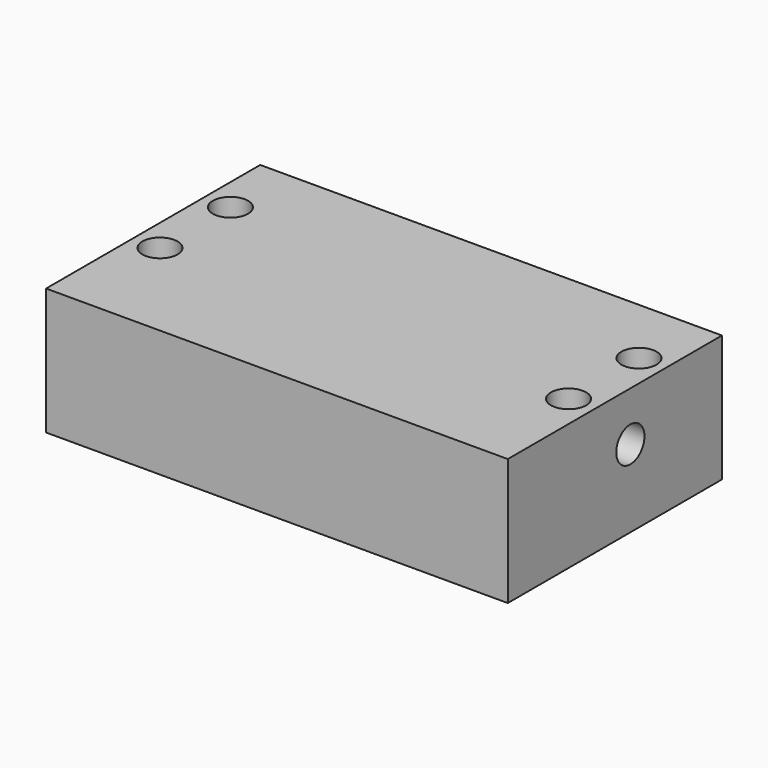
from build123d import *

# Parameters (mm, degrees)
F0_W     = 33.2994
F0_H     = 19.304
F1_DEPTH = 4.572
F2_R     = 1.27
F3_DEPTH = 2.54
F5_D     = 1.778
F5_DEPTH = 2.54
F5_TIP   = 0.5341650903
F8_R     = 1.27
F9_DEPTH = 9.145


# Not quite as in the source:
# - a pattern or mirror of a feature is missing from the dataset's text; its kind, count and spacing are read off the source's solid


with BuildPart() as f1:
    # F0 (on Top) → F1 (new body, symmetric)
    with BuildSketch(Plane.XY):
        Rectangle(F0_W, F0_H)
    extrude(amount=F1_DEPTH, both=True)

    # F2 (on face) → F3 (cut)
    with BuildSketch(Plane(origin=(-16.6497, 0, 0), x_dir=(0, -1, 0), z_dir=(-1, 0, 0))):
        with Locations((-1.397, 1.016)):
            Circle(F2_R)
    f3 = extrude(amount=-F3_DEPTH, mode=Mode.SUBTRACT)

    # F3_copies: F3 across plane
    add(f3.mirror(Plane(origin=(0, 0, 0), x_dir=(0, 0, 1), z_dir=(1, 0, 0))), mode=Mode.SUBTRACT)

    # F5
    with Locations(Plane(origin=(0, 0, -4.572), x_dir=(1, 0, 0), z_dir=(0, 0, -1))):
        with Locations((10.9347, -7.112), (10.9347, 7.112), (-10.9347, -7.112), (-10.9347, 7.112)):
            Hole(F5_D / 2, depth=F5_DEPTH)
            with Locations((0, 0, -(F5_DEPTH + F5_TIP / 2))):  # 118° drill point
                Cone(0, F5_D / 2, F5_TIP, mode=Mode.SUBTRACT)

    # F8 (on face) → F9 (cut, through all)
    with BuildSketch(Plane(origin=(0, 0, -4.572), x_dir=(1, 0, 0), z_dir=(0, 0, -1))):
        with Locations((-14.732, 1.778)):
            Circle(F8_R)
        with Locations((-14.732, -4.572)):
            Circle(F8_R)
        with Locations((14.732, 1.778)):
            Circle(F8_R)
        with Locations((14.732, -4.572)):
            Circle(F8_R)
    extrude(amount=-F9_DEPTH, mode=Mode.SUBTRACT)


solid = f1.part
